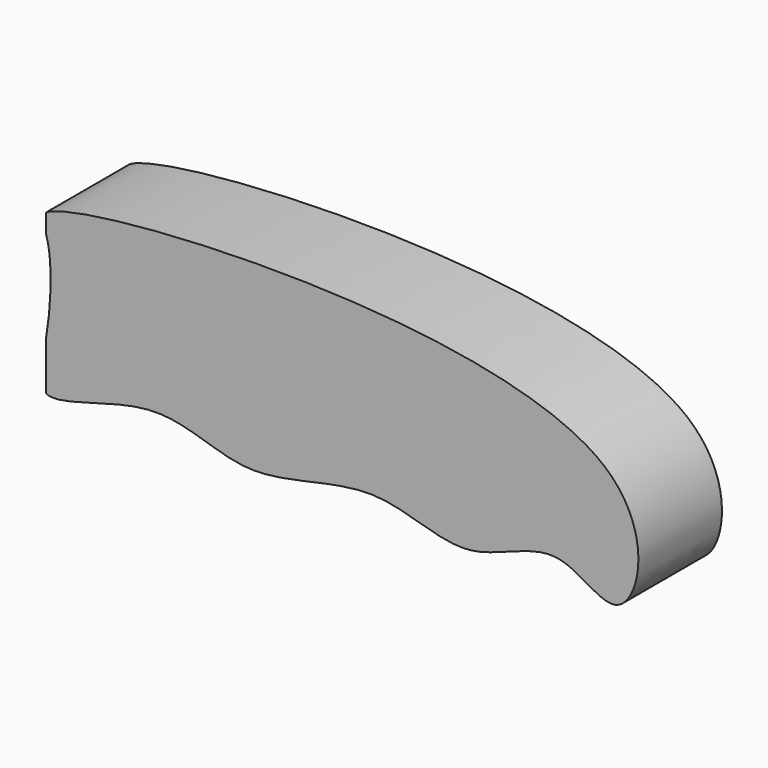
from build123d import *

# Parameters (mm, degrees)
F1_DEPTH = 11.43


# Not quite as in the source:
# - a feature of the source that left no trace in its solid (it failed there, or was rolled back) is left out


with BuildPart() as f1:
    # F0 (on Front) → F1 (new body)
    with BuildSketch(Plane.XZ):
        with BuildLine():
            add(Edge.make_bspline(
                [(-35.8184315264, -7.6753781177), (-34.1867990271, -8.5073013491), (-23.3050262159, -3.1679650902), (-13.9048580172, -9.8784881783), (0.1316174676, -3.6687063258), (10.2309447924, -9.9842260256), (20.0612737793, -2.6748573323), (28.0172360182, -11.955687996), (34.1409450761, 16.255689947), (-31.1984162209, 12.6926607697), (-35.8184315264, 9.7686629742)],
                knots=[0, 0, 0, 0, 0.089979129, 0.1781652343, 0.2757094492, 0.3618933063, 0.4456564152, 0.5151675526, 0.6099891246, 0.8170248264, 0.8170248264, 0.8170248264, 0.8170248264], degree=3))
            Line((-35.8184315264, 9.7686629742), (-35.8184315264, 7.6753781177))
            add(Edge.make_bspline(
                [(-35.8184315264, 7.6753781177), (-35.0854948786, 5.4968902562), (-35.2258651996, 1.2155212089), (-35.8184315264, -2.3258721922)],
                knots=[0.8552687604, 0.8552687604, 0.8552687604, 0.8552687604, 0.9388628442, 0.9388628442, 0.9388628442, 0.9388628442], degree=3))
            Line((-35.8184315264, -2.3258721922), (-35.8184315264, -7.6753781177))
        make_face()
    extrude(amount=-F1_DEPTH)


solid = f1.part
